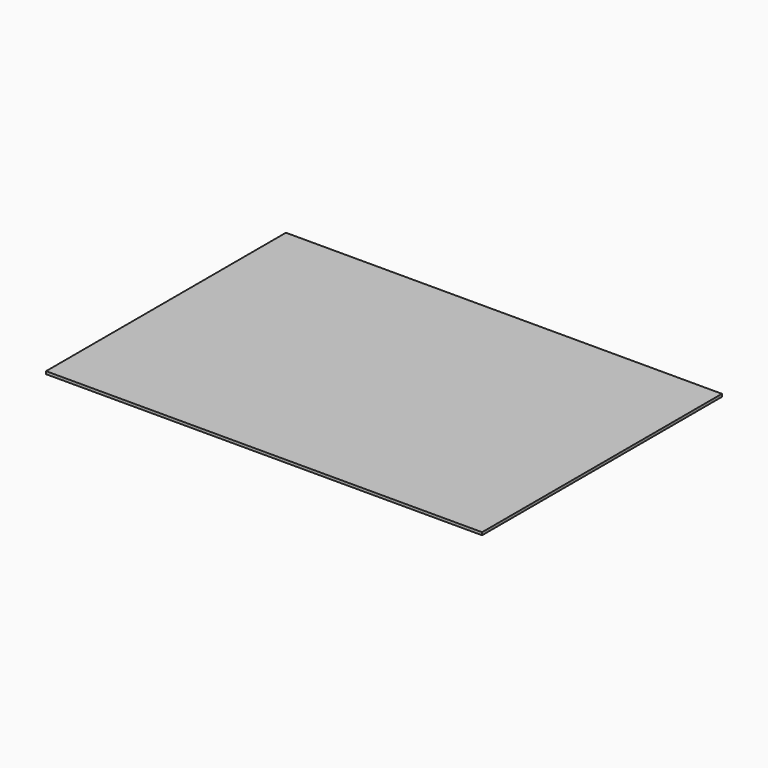
from build123d import *

# Parameters (mm, degrees)
F0_W     = 762
F0_H     = 523.875
F1_DEPTH = 4.7625


# Not quite as in the source:
# - a length typed as a fraction of an inch, garbled in the dataset ("3 / 203.2 mm" for 3/8 in), is restored


with BuildPart() as f1:
    # F0 (on Top) → F1 (new body)
    with BuildSketch(Plane.XY):
        with Locations((-533.7140479332, 5.7780072093)):
            Rectangle(F0_W, F0_H)
    extrude(amount=-F1_DEPTH)


solid = f1.part
